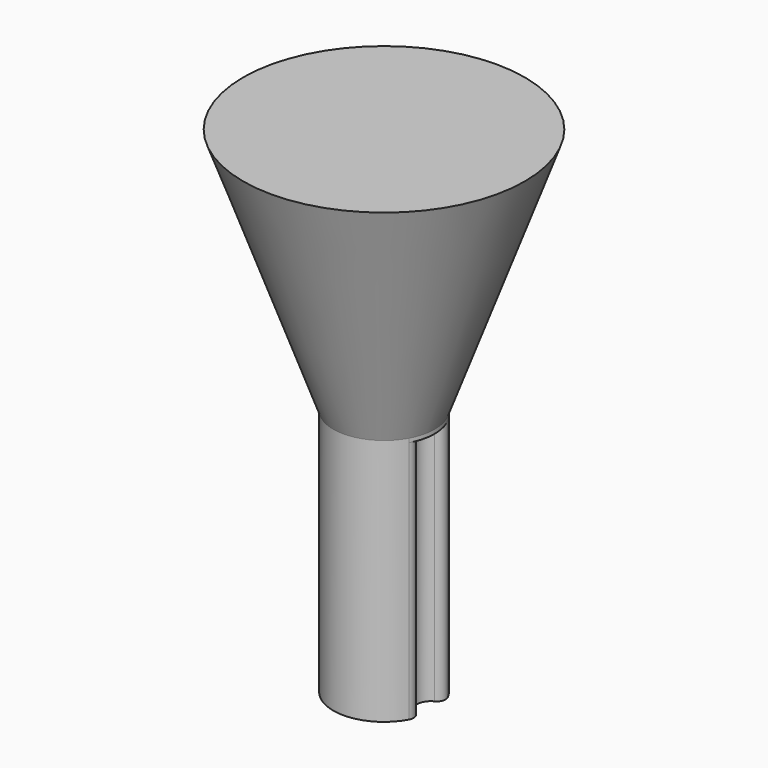
from build123d import *
from build123d import SkipClean  # not in build123d's __all__

# Parameters (mm, degrees)
F1_DEPTH = 12.7
F2_R     = 2.6
F3_DEPTH = 12.7
F3_TAPER = -20
F6_DEPTH = 0.2


with BuildPart() as f1:
    # F0 (on Top) → F1 (new body)
    with BuildSketch(Plane.XY):
        with BuildLine():
            ThreePointArc((2.0857885615, 0.6255167239), (2.315451032, 0.8961675136), (2.2801491146, 1.2493678462))
            ThreePointArc((2.2801491146, 1.2493678462), (-2.6, 0), (2.2801491146, -1.2493678462))
            ThreePointArc((2.2801491146, -1.2493678462), (2.315451032, -0.8961675136), (2.0857885615, -0.6255167239))
            ThreePointArc((2.0857885615, -0.6255167239), (1.7, 0), (2.0857885615, 0.6255167239))
        make_face()
    extrude(amount=-F1_DEPTH)

    # F2 (on Top) → F3 (join)
    with BuildSketch(Plane.XY):
        Circle(F2_R)
    extrude(amount=F3_DEPTH, taper=F3_TAPER)

    # F5 (on face) → F6 (join)
    with BuildSketch(Plane(origin=(0, 0, 0), x_dir=(1, 0, 0), z_dir=(0, 0, -1))):
        with BuildLine():
            ThreePointArc((2.2801491146, 1.2493678462), (2.315451032, 0.8961675136), (2.0857885615, 0.6255167239))
            ThreePointArc((2.0857885615, 0.6255167239), (1.7, 0), (2.0857885615, -0.6255167239))
            ThreePointArc((2.0857885615, -0.6255167239), (2.315451032, -0.8961675136), (2.2801491146, -1.2493678462))
            ThreePointArc((2.2801491146, -1.2493678462), (2.6, 0), (2.2801491146, 1.2493678462))
        make_face()
    with SkipClean():  # cleaning this boolean's faces spoils the solid; the shape is the same uncleaned
        extrude(amount=F6_DEPTH)


solid = f1.part
